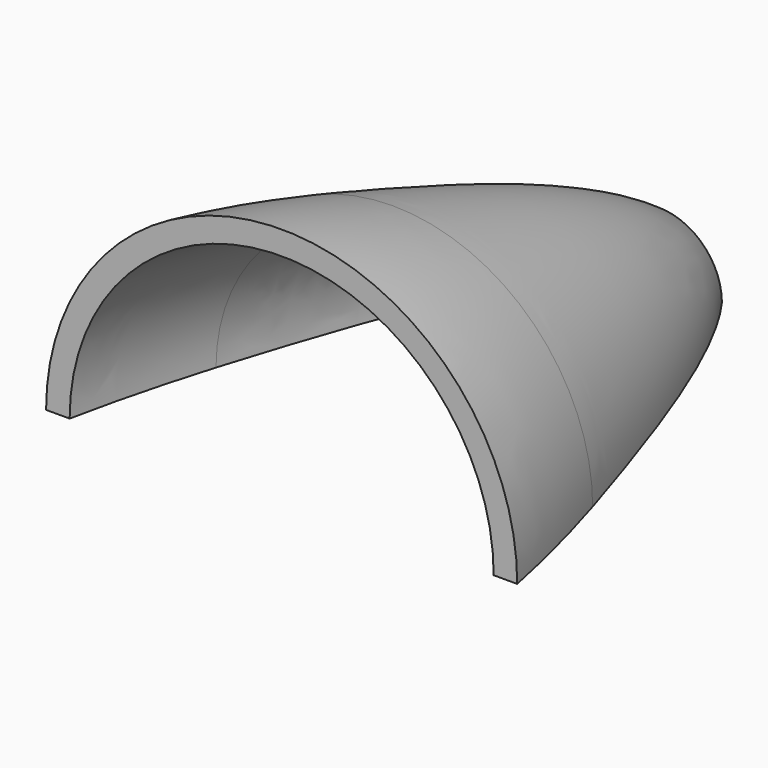
from build123d import *

# Parameters (mm, degrees)
F1_ANGLE = 180


# Not quite as in the source:
# - the dataset's text gives a spline's control points without its knots; the knots are read off the source's solid


with BuildPart() as f1:
    # F0 (on Top) → F1 (revolve)
    with BuildSketch(Plane.XY):
        with BuildLine():
            Line((-15.0155171111, 69.1660211089), (-41.8962485401, 69.1660211089))
            Line((-41.8962485401, 69.1660211089), (-41.8963717975, 59.1659390384))
            Line((-41.8963717975, 59.1659390384), (-20.2472324434, 59.1659390491))
            add(Edge.make_bspline(
                [(33.1035238522, -71.9149671498), (32.1956039275, -68.8975063653), (30.6294745703, -63.7909684), (28.3196130402, -56.4725000911), (26.2505964512, -50.0519807984), (24.0990817026, -43.5000705854), (21.8647786098, -36.8081776409), (19.5529594243, -30.0145868681), (16.3683569347, -20.8591029876), (12.2012714526, -9.3103100361), (6.9186898701, 4.4674267501), (-0.4742289291, 22.3935878339), (-8.3508677217, 39.1456078716), (-15.719087441, 52.1661135478), (-19.0226095104, 57.3411254378), (-20.2472324434, 59.1659390491)],
                knots=[0.3286112864, 0.3286112864, 0.3286112864, 0.3286112864, 0.375, 0.40625, 0.4375, 0.46875, 0.5, 0.53125, 0.5625, 0.625, 0.6875, 0.75, 0.875, 0.9375, 0.9742015542, 0.9742015542, 0.9742015542, 0.9742015542], degree=3))
            Line((33.1035238522, -71.9149671498), (42.9852085247, -71.9149671498))
            add(Edge.make_bspline(
                [(42.9852085247, -71.9149671498), (39.9590182528, -62.0062274912), (25.1654617563, -16.1855840824), (4.2573580541, 42.5444841716), (-15.0155171111, 69.1660211089)],
                knots=[0.3152642845, 0.3152642845, 0.3152642845, 0.3152642845, 0.4687726258, 1, 1, 1, 1], degree=3))
        make_face()
        with BuildLine():
            add(Edge.make_bspline(
                [(58.1037514599, -130.8339788911), (54.1906296951, -111.0809956414), (49.2001783618, -92.2648171488), (42.9852085247, -71.9149671498)],
                knots=[0, 0, 0, 0, 0.3152642845, 0.3152642845, 0.3152642845, 0.3152642845], degree=3))
            Line((42.9852085247, -71.9149671498), (33.1035238522, -71.9149671498))
            add(Edge.make_bspline(
                [(48.1037514599, -130.8339788911), (46.7078713802, -123.9406660172), (44.3454121428, -113.2929426353), (40.6901923565, -98.7187159107), (37.5318209869, -87.037434), (34.9410521612, -78.0565994752), (33.4188539578, -72.9629629054), (33.1035238522, -71.9149671498)],
                knots=[0.0128290388, 0.0128290388, 0.0128290388, 0.0128290388, 0.125, 0.1875, 0.25, 0.3125, 0.3286112864, 0.3286112864, 0.3286112864, 0.3286112864], degree=3))
            Line((48.1037514599, -130.8339788911), (58.1037514599, -130.8339788911))
        make_face()
    revolve(axis=Axis((-41.8963717672, -2.0099732555, 0), (5e-10, -1, 0)), revolution_arc=F1_ANGLE)


solid = f1.part
